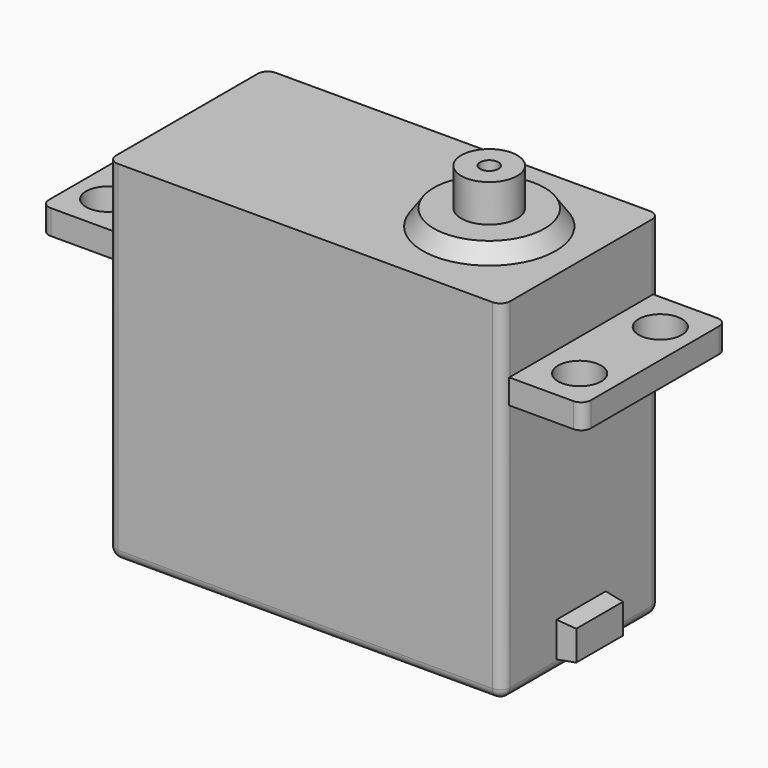
from build123d import *

# Parameters (mm, degrees)
F0_W           = 40.64
F0_H           = 20.32
F1_DEPTH       = 36.068
F2_W           = 6.35
F2_H           = 3.6068
F4_W           = 6.0198
F4_H           = 3.0734
F7_R           = 2.2225
F8_DEPTH       = 2.54
F9_R           = 6.858
F11_R          = 5.7023
F13_T1_DEPTH   = 38.608
F13_T3_DEPTH   = 18.288
F13_S7_W       = 1.016
F13_S7_H       = 1.016
F13_T8_DEPTH   = 1.016
F13_S13_W      = 1.016
F13_S13_H      = 1.016
F13_T14_DEPTH  = 1.016
F13_S19_W      = 1.016
F13_S19_H      = 1.016
F13_T20_DEPTH  = 1.016
F13_S25_W      = 1.016
F13_S25_H      = 1.016
F13_T26_DEPTH  = 1.016
F13_T32_DEPTH  = 37.592
F13_T38_DEPTH  = 37.592
F13_T44_DEPTH  = 37.592
F13_T51_DEPTH  = 37.592
F13_T57_DEPTH  = 37.592
F13_T63_DEPTH  = 37.592
F13_T69_DEPTH  = 37.592
F13_T75_DEPTH  = 37.592
F13_T82_DEPTH  = 37.592
F13_T88_DEPTH  = 37.592
F13_T94_DEPTH  = 37.592
F13_T100_DEPTH = 37.592
F13_T106_DEPTH = 37.592
F13_T113_DEPTH = 37.592
F13_T119_DEPTH = 37.592
F13_T125_DEPTH = 37.592
F13_T131_DEPTH = 37.592
F13_T137_DEPTH = 37.592
F13_T144_DEPTH = 37.592
F13_T150_DEPTH = 37.592
F14_R          = 2.8829
F14_R_2        = 0.9398
F15_DEPTH      = 3.8608


# Not quite as in the source:
# - a fillet or chamfer that OpenCascade refuses, or shapes differently, is made with other operations: its cross-section is extruded or revolved along the edge and cut away or added


with BuildPart() as f1:
    # F0 (on Top) → F1 (new body)
    with BuildSketch(Plane.XY):
        Rectangle(F0_W, F0_H)
    extrude(amount=F1_DEPTH)

    # F2 (on face) → F5 section 0
    with BuildSketch(Plane.YZ.offset(20.32)):
        with Locations((0, 2.9464)):
            Rectangle(F2_W, F2_H)
    # F4 (on offset) → F5 section 1
    with BuildSketch(Plane.YZ.offset(22.225)):
        with Locations((0, 2.9464)):
            Rectangle(F4_W, F4_H)
    loft()

    # F7 (on offset) → F8 (join)
    with BuildSketch(Plane.XY.offset(29.21)):
        with BuildLine():
            ThreePointArc((-27.94, -8.255), (-27.6424204897, -8.9734204897), (-26.924, -9.271))
            Line((-26.924, -9.271), (-20.32, -9.271))
            Line((-20.32, -9.271), (-20.32, 9.271))
            Line((-20.32, 9.271), (-26.924, 9.271))
            ThreePointArc((-26.924, 9.271), (-27.6424204897, 8.9734204897), (-27.94, 8.255))
            Line((-27.94, 8.255), (-27.94, -8.255))
        make_face()
        with Locations((-24.3205, -5.1943)):
            Circle(F7_R, mode=Mode.SUBTRACT)
        with Locations((-24.3205, 5.1943)):
            Circle(F7_R, mode=Mode.SUBTRACT)
        with BuildLine():
            ThreePointArc((27.94, 8.255), (27.6424204897, 8.9734204897), (26.924, 9.271))
            Line((26.924, 9.271), (20.32, 9.271))
            Line((20.32, 9.271), (20.32, -9.271))
            Line((20.32, -9.271), (26.924, -9.271))
            ThreePointArc((26.924, -9.271), (27.6424204897, -8.9734204897), (27.94, -8.255))
            Line((27.94, -8.255), (27.94, 8.255))
        make_face()
        with Locations((24.3205, -5.1943)):
            Circle(F7_R, mode=Mode.SUBTRACT)
        with Locations((24.3205, 5.1943)):
            Circle(F7_R, mode=Mode.SUBTRACT)
    extrude(amount=-F8_DEPTH)

    # F9 (on face) → F12 section 0
    with BuildSketch(Plane.XY.offset(36.068)):
        with Locations((10.8458, 0)):
            Circle(F9_R)
    # F11 (on offset) → F12 section 1
    with BuildSketch(Plane.XY.offset(37.719)):
        with Locations((10.8458, 0)):
            Circle(F11_R)
    loft()

    # F13: fillet of radius 1.016 on 8 edges, made by hand

    # F13_s2 → F13_t1 (cut)
    with BuildSketch(Plane.YZ.offset(-19.304)):
        with BuildLine():
            ThreePointArc((-10.16, 1.016), (-9.8624204897, 0.2975795103), (-9.144, 0))
            Line((-9.144, 0), (-10.16, 0))
            Line((-10.16, 0), (-10.16, 1.016))
        make_face()
        with BuildLine():
            ThreePointArc((9.144, 0), (9.8624204897, 0.2975795103), (10.16, 1.016))
            Line((10.16, 1.016), (10.16, 0))
            Line((10.16, 0), (9.144, 0))
        make_face()
    extrude(amount=F13_T1_DEPTH, mode=Mode.SUBTRACT)

    # F13_s4 → F13_t3 (cut)
    with BuildSketch(Plane.XZ.offset(-9.144)):
        with BuildLine():
            ThreePointArc((20.32, 1.016), (20.0224204897, 0.2975795103), (19.304, 0))
            Line((19.304, 0), (20.32, 0))
            Line((20.32, 0), (20.32, 1.016))
        make_face()
        with BuildLine():
            ThreePointArc((-19.304, 0), (-20.0224204897, 0.2975795103), (-20.32, 1.016))
            Line((-20.32, 1.016), (-20.32, 0))
            Line((-20.32, 0), (-19.304, 0))
        make_face()
    extrude(amount=F13_T3_DEPTH, mode=Mode.SUBTRACT)


with BuildPart() as f13_tool6:
    # F13_s7 → F13_t8 (new body)
    with BuildSketch(Plane.YZ.offset(19.304)):
        with Locations((-9.652, 0.508)):
            Rectangle(F13_S7_W, F13_S7_H)
    extrude(amount=F13_T8_DEPTH)

    # F13_s9 → F13_t10 (revolve, cut)
    with BuildSketch(Plane(origin=(19.304, -9.144, 1.016), x_dir=(0, 0.7071067812, 0.7071067812), z_dir=(0, 0.7071067812, -0.7071067812))):
        with BuildLine():
            ThreePointArc((0, -1.016), (1.016, 0), (0, 1.016))
            Line((0, 1.016), (0, -1.016))
        make_face()
    revolve(axis=Axis((19.304, -9.144, 1.016), (1, 0, 0)), mode=Mode.SUBTRACT)


with BuildPart() as f1_1:
    add(f1.part)

    # F13_t5: cut F13_tool6
    add(f13_tool6.part, mode=Mode.SUBTRACT)


with BuildPart() as f13_tool12:
    # F13_s13 → F13_t14 (new body)
    with BuildSketch(Plane.YZ.offset(19.304)):
        with Locations((9.652, 0.508)):
            Rectangle(F13_S13_W, F13_S13_H)
    extrude(amount=F13_T14_DEPTH)

    # F13_s15 → F13_t16 (revolve, cut)
    with BuildSketch(Plane(origin=(19.304, 9.144, 1.016), x_dir=(0, -0.7071067812, 0.7071067812), z_dir=(0, 0.7071067812, 0.7071067812))):
        with BuildLine():
            ThreePointArc((0, -1.016), (1.016, 0), (0, 1.016))
            Line((0, 1.016), (0, -1.016))
        make_face()
    revolve(axis=Axis((19.304, 9.144, 1.016), (1, 0, 0)), mode=Mode.SUBTRACT)


with BuildPart() as f1_2:
    add(f1_1.part)

    # F13_t11: cut F13_tool12
    add(f13_tool12.part, mode=Mode.SUBTRACT)


with BuildPart() as f13_tool18:
    # F13_s19 → F13_t20 (new body)
    with BuildSketch(Plane.XY.offset(1.016)):
        with Locations((-19.812, 9.652)):
            Rectangle(F13_S19_W, F13_S19_H)
    extrude(amount=-F13_T20_DEPTH)

    # F13_s21 → F13_t22 (revolve, cut)
    with BuildSketch(Plane(origin=(-19.304, 9.144, 1.016), x_dir=(0.7071067812, -0.7071067812, 0), z_dir=(0.7071067812, 0.7071067812, 0))):
        with BuildLine():
            ThreePointArc((0, -1.016), (1.016, 0), (0, 1.016))
            Line((0, 1.016), (0, -1.016))
        make_face()
    revolve(axis=Axis((-19.304, 9.144, 1.016), (0, 0, -1)), mode=Mode.SUBTRACT)


with BuildPart() as f1_3:
    add(f1_2.part)

    # F13_t17: cut F13_tool18
    add(f13_tool18.part, mode=Mode.SUBTRACT)


with BuildPart() as f13_tool24:
    # F13_s25 → F13_t26 (new body)
    with BuildSketch(Plane.XZ.offset(9.144)):
        with Locations((-19.812, 0.508)):
            Rectangle(F13_S25_W, F13_S25_H)
    extrude(amount=F13_T26_DEPTH)

    # F13_s27 → F13_t28 (revolve, cut)
    with BuildSketch(Plane(origin=(-19.304, -9.144, 1.016), x_dir=(0.7071067812, 0, 0.7071067812), z_dir=(0.7071067812, 0, -0.7071067812))):
        with BuildLine():
            ThreePointArc((0, -1.016), (1.016, 0), (0, 1.016))
            Line((0, 1.016), (0, -1.016))
        make_face()
    revolve(axis=Axis((-19.304, -9.144, 1.016), (0, -1, 0)), mode=Mode.SUBTRACT)


with BuildPart() as f1_4:
    add(f1_3.part)

    # F13_t23: cut F13_tool24
    add(f13_tool24.part, mode=Mode.SUBTRACT)


with BuildPart() as f13_tool30:
    # F13_s31 → F13_t32 (new body)
    with BuildSketch(Plane.XY.offset(1.016)):
        with BuildLine():
            ThreePointArc((20.32, -9.144), (20.0224204897, -9.8624204897), (19.304, -10.16))
            Line((19.304, -10.16), (20.32, -10.16))
            Line((20.32, -10.16), (20.32, -9.144))
        make_face()
    extrude(amount=F13_T32_DEPTH)

    split(bisect_by=Plane.XY.offset(26.67), keep=Keep.BOTTOM)

    split(bisect_by=Plane.XZ.offset(9.271), keep=Keep.BOTTOM)


with BuildPart() as f1_5:
    add(f1_4.part)

    # F13_t29: cut F13_tool30
    add(f13_tool30.part, mode=Mode.SUBTRACT)


with BuildPart() as f13_tool36:
    # F13_s37 → F13_t38 (new body)
    with BuildSketch(Plane.XY.offset(1.016)):
        with BuildLine():
            ThreePointArc((20.32, -9.144), (20.0224204897, -9.8624204897), (19.304, -10.16))
            Line((19.304, -10.16), (20.32, -10.16))
            Line((20.32, -10.16), (20.32, -9.144))
        make_face()
    extrude(amount=F13_T38_DEPTH)

    split(bisect_by=Plane.XY.offset(26.67), keep=Keep.BOTTOM)

    split(bisect_by=Plane.XZ.offset(9.271), keep=Keep.TOP)


with BuildPart() as f1_6:
    add(f1_5.part)

    # F13_t35: cut F13_tool36
    add(f13_tool36.part, mode=Mode.SUBTRACT)


with BuildPart() as f13_tool42:
    # F13_s43 → F13_t44 (new body)
    with BuildSketch(Plane.XY.offset(1.016)):
        with BuildLine():
            ThreePointArc((20.32, -9.144), (20.0224204897, -9.8624204897), (19.304, -10.16))
            Line((19.304, -10.16), (20.32, -10.16))
            Line((20.32, -10.16), (20.32, -9.144))
        make_face()
    extrude(amount=F13_T44_DEPTH)

    split(bisect_by=Plane.XY.offset(26.67), keep=Keep.TOP)

    split(bisect_by=Plane.XZ.offset(9.271), keep=Keep.TOP)

    split(bisect_by=Plane.XY.offset(29.21), keep=Keep.BOTTOM)


with BuildPart() as f1_7:
    add(f1_6.part)

    # F13_t41: cut F13_tool42
    add(f13_tool42.part, mode=Mode.SUBTRACT)


with BuildPart() as f13_tool49:
    # F13_s50 → F13_t51 (new body)
    with BuildSketch(Plane.XY.offset(1.016)):
        with BuildLine():
            ThreePointArc((20.32, -9.144), (20.0224204897, -9.8624204897), (19.304, -10.16))
            Line((19.304, -10.16), (20.32, -10.16))
            Line((20.32, -10.16), (20.32, -9.144))
        make_face()
    extrude(amount=F13_T51_DEPTH)

    split(bisect_by=Plane.XZ.offset(9.271), keep=Keep.BOTTOM)

    split(bisect_by=Plane.XY.offset(29.21), keep=Keep.TOP)


with BuildPart() as f1_8:
    add(f1_7.part)

    # F13_t48: cut F13_tool49
    add(f13_tool49.part, mode=Mode.SUBTRACT)


with BuildPart() as f13_tool55:
    # F13_s56 → F13_t57 (new body)
    with BuildSketch(Plane.XY.offset(1.016)):
        with BuildLine():
            ThreePointArc((20.32, -9.144), (20.0224204897, -9.8624204897), (19.304, -10.16))
            Line((19.304, -10.16), (20.32, -10.16))
            Line((20.32, -10.16), (20.32, -9.144))
        make_face()
    extrude(amount=F13_T57_DEPTH)

    split(bisect_by=Plane.XZ.offset(9.271), keep=Keep.TOP)

    split(bisect_by=Plane.XY.offset(29.21), keep=Keep.TOP)


with BuildPart() as f1_9:
    add(f1_8.part)

    # F13_t54: cut F13_tool55
    add(f13_tool55.part, mode=Mode.SUBTRACT)


with BuildPart() as f13_tool61:
    # F13_s62 → F13_t63 (new body)
    with BuildSketch(Plane.XY.offset(1.016)):
        with BuildLine():
            ThreePointArc((20.32, 9.144), (20.0224204897, 9.8624204897), (19.304, 10.16))
            Line((19.304, 10.16), (20.32, 10.16))
            Line((20.32, 10.16), (20.32, 9.144))
        make_face()
    extrude(amount=F13_T63_DEPTH)

    split(bisect_by=Plane.XZ.offset(-9.271), keep=Keep.TOP)

    split(bisect_by=Plane.XY.offset(26.67), keep=Keep.BOTTOM)


with BuildPart() as f1_10:
    add(f1_9.part)

    # F13_t60: cut F13_tool61
    add(f13_tool61.part, mode=Mode.SUBTRACT)


with BuildPart() as f13_tool67:
    # F13_s68 → F13_t69 (new body)
    with BuildSketch(Plane.XY.offset(1.016)):
        with BuildLine():
            ThreePointArc((20.32, 9.144), (20.0224204897, 9.8624204897), (19.304, 10.16))
            Line((19.304, 10.16), (20.32, 10.16))
            Line((20.32, 10.16), (20.32, 9.144))
        make_face()
    extrude(amount=F13_T69_DEPTH)

    split(bisect_by=Plane.XZ.offset(-9.271), keep=Keep.BOTTOM)

    split(bisect_by=Plane.XY.offset(26.67), keep=Keep.BOTTOM)


with BuildPart() as f1_11:
    add(f1_10.part)

    # F13_t66: cut F13_tool67
    add(f13_tool67.part, mode=Mode.SUBTRACT)


with BuildPart() as f13_tool73:
    # F13_s74 → F13_t75 (new body)
    with BuildSketch(Plane.XY.offset(1.016)):
        with BuildLine():
            ThreePointArc((20.32, 9.144), (20.0224204897, 9.8624204897), (19.304, 10.16))
            Line((19.304, 10.16), (20.32, 10.16))
            Line((20.32, 10.16), (20.32, 9.144))
        make_face()
    extrude(amount=F13_T75_DEPTH)

    split(bisect_by=Plane.XZ.offset(-9.271), keep=Keep.BOTTOM)

    split(bisect_by=Plane.XY.offset(26.67), keep=Keep.TOP)

    split(bisect_by=Plane.XY.offset(29.21), keep=Keep.BOTTOM)


with BuildPart() as f1_12:
    add(f1_11.part)

    # F13_t72: cut F13_tool73
    add(f13_tool73.part, mode=Mode.SUBTRACT)


with BuildPart() as f13_tool80:
    # F13_s81 → F13_t82 (new body)
    with BuildSketch(Plane.XY.offset(1.016)):
        with BuildLine():
            ThreePointArc((20.32, 9.144), (20.0224204897, 9.8624204897), (19.304, 10.16))
            Line((19.304, 10.16), (20.32, 10.16))
            Line((20.32, 10.16), (20.32, 9.144))
        make_face()
    extrude(amount=F13_T82_DEPTH)

    split(bisect_by=Plane.XZ.offset(-9.271), keep=Keep.TOP)

    split(bisect_by=Plane.XY.offset(29.21), keep=Keep.TOP)


with BuildPart() as f1_13:
    add(f1_12.part)

    # F13_t79: cut F13_tool80
    add(f13_tool80.part, mode=Mode.SUBTRACT)


with BuildPart() as f13_tool86:
    # F13_s87 → F13_t88 (new body)
    with BuildSketch(Plane.XY.offset(1.016)):
        with BuildLine():
            ThreePointArc((20.32, 9.144), (20.0224204897, 9.8624204897), (19.304, 10.16))
            Line((19.304, 10.16), (20.32, 10.16))
            Line((20.32, 10.16), (20.32, 9.144))
        make_face()
    extrude(amount=F13_T88_DEPTH)

    split(bisect_by=Plane.XZ.offset(-9.271), keep=Keep.BOTTOM)

    split(bisect_by=Plane.XY.offset(29.21), keep=Keep.TOP)


with BuildPart() as f1_14:
    add(f1_13.part)

    # F13_t85: cut F13_tool86
    add(f13_tool86.part, mode=Mode.SUBTRACT)


with BuildPart() as f13_tool92:
    # F13_s93 → F13_t94 (new body)
    with BuildSketch(Plane.XY.offset(1.016)):
        with BuildLine():
            ThreePointArc((-19.304, 10.16), (-20.0224204897, 9.8624204897), (-20.32, 9.144))
            Line((-20.32, 9.144), (-20.32, 10.16))
            Line((-20.32, 10.16), (-19.304, 10.16))
        make_face()
    extrude(amount=F13_T94_DEPTH)

    split(bisect_by=Plane.XY.offset(26.67), keep=Keep.BOTTOM)

    split(bisect_by=Plane.XZ.offset(-9.271), keep=Keep.BOTTOM)


with BuildPart() as f1_15:
    add(f1_14.part)

    # F13_t91: cut F13_tool92
    add(f13_tool92.part, mode=Mode.SUBTRACT)


with BuildPart() as f13_tool98:
    # F13_s99 → F13_t100 (new body)
    with BuildSketch(Plane.XY.offset(1.016)):
        with BuildLine():
            ThreePointArc((-19.304, 10.16), (-20.0224204897, 9.8624204897), (-20.32, 9.144))
            Line((-20.32, 9.144), (-20.32, 10.16))
            Line((-20.32, 10.16), (-19.304, 10.16))
        make_face()
    extrude(amount=F13_T100_DEPTH)

    split(bisect_by=Plane.XY.offset(26.67), keep=Keep.BOTTOM)

    split(bisect_by=Plane.XZ.offset(-9.271), keep=Keep.TOP)


with BuildPart() as f1_16:
    add(f1_15.part)

    # F13_t97: cut F13_tool98
    add(f13_tool98.part, mode=Mode.SUBTRACT)


with BuildPart() as f13_tool104:
    # F13_s105 → F13_t106 (new body)
    with BuildSketch(Plane.XY.offset(1.016)):
        with BuildLine():
            ThreePointArc((-19.304, 10.16), (-20.0224204897, 9.8624204897), (-20.32, 9.144))
            Line((-20.32, 9.144), (-20.32, 10.16))
            Line((-20.32, 10.16), (-19.304, 10.16))
        make_face()
    extrude(amount=F13_T106_DEPTH)

    split(bisect_by=Plane.XY.offset(26.67), keep=Keep.TOP)

    split(bisect_by=Plane.XZ.offset(-9.271), keep=Keep.BOTTOM)

    split(bisect_by=Plane.XY.offset(29.21), keep=Keep.BOTTOM)


with BuildPart() as f1_17:
    add(f1_16.part)

    # F13_t103: cut F13_tool104
    add(f13_tool104.part, mode=Mode.SUBTRACT)


with BuildPart() as f13_tool111:
    # F13_s112 → F13_t113 (new body)
    with BuildSketch(Plane.XY.offset(1.016)):
        with BuildLine():
            ThreePointArc((-19.304, 10.16), (-20.0224204897, 9.8624204897), (-20.32, 9.144))
            Line((-20.32, 9.144), (-20.32, 10.16))
            Line((-20.32, 10.16), (-19.304, 10.16))
        make_face()
    extrude(amount=F13_T113_DEPTH)

    split(bisect_by=Plane.XZ.offset(-9.271), keep=Keep.BOTTOM)

    split(bisect_by=Plane.XY.offset(29.21), keep=Keep.TOP)


with BuildPart() as f1_18:
    add(f1_17.part)

    # F13_t110: cut F13_tool111
    add(f13_tool111.part, mode=Mode.SUBTRACT)


with BuildPart() as f13_tool117:
    # F13_s118 → F13_t119 (new body)
    with BuildSketch(Plane.XY.offset(1.016)):
        with BuildLine():
            ThreePointArc((-19.304, 10.16), (-20.0224204897, 9.8624204897), (-20.32, 9.144))
            Line((-20.32, 9.144), (-20.32, 10.16))
            Line((-20.32, 10.16), (-19.304, 10.16))
        make_face()
    extrude(amount=F13_T119_DEPTH)

    split(bisect_by=Plane.XZ.offset(-9.271), keep=Keep.TOP)

    split(bisect_by=Plane.XY.offset(29.21), keep=Keep.TOP)


with BuildPart() as f1_19:
    add(f1_18.part)

    # F13_t116: cut F13_tool117
    add(f13_tool117.part, mode=Mode.SUBTRACT)


with BuildPart() as f13_tool123:
    # F13_s124 → F13_t125 (new body)
    with BuildSketch(Plane.XY.offset(1.016)):
        with BuildLine():
            ThreePointArc((-19.304, -10.16), (-20.0224204897, -9.8624204897), (-20.32, -9.144))
            Line((-20.32, -9.144), (-20.32, -10.16))
            Line((-20.32, -10.16), (-19.304, -10.16))
        make_face()
    extrude(amount=F13_T125_DEPTH)

    split(bisect_by=Plane.XZ.offset(9.271), keep=Keep.TOP)

    split(bisect_by=Plane.XY.offset(26.67), keep=Keep.BOTTOM)


with BuildPart() as f1_20:
    add(f1_19.part)

    # F13_t122: cut F13_tool123
    add(f13_tool123.part, mode=Mode.SUBTRACT)


with BuildPart() as f13_tool129:
    # F13_s130 → F13_t131 (new body)
    with BuildSketch(Plane.XY.offset(1.016)):
        with BuildLine():
            ThreePointArc((-19.304, -10.16), (-20.0224204897, -9.8624204897), (-20.32, -9.144))
            Line((-20.32, -9.144), (-20.32, -10.16))
            Line((-20.32, -10.16), (-19.304, -10.16))
        make_face()
    extrude(amount=F13_T131_DEPTH)

    split(bisect_by=Plane.XZ.offset(9.271), keep=Keep.BOTTOM)

    split(bisect_by=Plane.XY.offset(26.67), keep=Keep.BOTTOM)


with BuildPart() as f1_21:
    add(f1_20.part)

    # F13_t128: cut F13_tool129
    add(f13_tool129.part, mode=Mode.SUBTRACT)


with BuildPart() as f13_tool135:
    # F13_s136 → F13_t137 (new body)
    with BuildSketch(Plane.XY.offset(1.016)):
        with BuildLine():
            ThreePointArc((-19.304, -10.16), (-20.0224204897, -9.8624204897), (-20.32, -9.144))
            Line((-20.32, -9.144), (-20.32, -10.16))
            Line((-20.32, -10.16), (-19.304, -10.16))
        make_face()
    extrude(amount=F13_T137_DEPTH)

    split(bisect_by=Plane.XZ.offset(9.271), keep=Keep.TOP)

    split(bisect_by=Plane.XY.offset(26.67), keep=Keep.TOP)

    split(bisect_by=Plane.XY.offset(29.21), keep=Keep.BOTTOM)


with BuildPart() as f1_22:
    add(f1_21.part)

    # F13_t134: cut F13_tool135
    add(f13_tool135.part, mode=Mode.SUBTRACT)


with BuildPart() as f13_tool142:
    # F13_s143 → F13_t144 (new body)
    with BuildSketch(Plane.XY.offset(1.016)):
        with BuildLine():
            ThreePointArc((-19.304, -10.16), (-20.0224204897, -9.8624204897), (-20.32, -9.144))
            Line((-20.32, -9.144), (-20.32, -10.16))
            Line((-20.32, -10.16), (-19.304, -10.16))
        make_face()
    extrude(amount=F13_T144_DEPTH)

    split(bisect_by=Plane.XZ.offset(9.271), keep=Keep.TOP)

    split(bisect_by=Plane.XY.offset(29.21), keep=Keep.TOP)


with BuildPart() as f1_23:
    add(f1_22.part)

    # F13_t141: cut F13_tool142
    add(f13_tool142.part, mode=Mode.SUBTRACT)


with BuildPart() as f13_tool148:
    # F13_s149 → F13_t150 (new body)
    with BuildSketch(Plane.XY.offset(1.016)):
        with BuildLine():
            ThreePointArc((-19.304, -10.16), (-20.0224204897, -9.8624204897), (-20.32, -9.144))
            Line((-20.32, -9.144), (-20.32, -10.16))
            Line((-20.32, -10.16), (-19.304, -10.16))
        make_face()
    extrude(amount=F13_T150_DEPTH)

    split(bisect_by=Plane.XZ.offset(9.271), keep=Keep.BOTTOM)

    split(bisect_by=Plane.XY.offset(29.21), keep=Keep.TOP)


with BuildPart() as f1_24:
    add(f1_23.part)

    # F13_t147: cut F13_tool148
    add(f13_tool148.part, mode=Mode.SUBTRACT)


with BuildPart() as f15:
    # F14 (on face) → F15 (new body)
    with BuildSketch(Plane.XY.offset(37.719)):
        with Locations((10.8458, 0)):
            Circle(F14_R)
        with Locations((10.8458, 0)):
            Circle(F14_R_2, mode=Mode.SUBTRACT)
    extrude(amount=F15_DEPTH)


solid = Compound([f1_24.part, f15.part])
